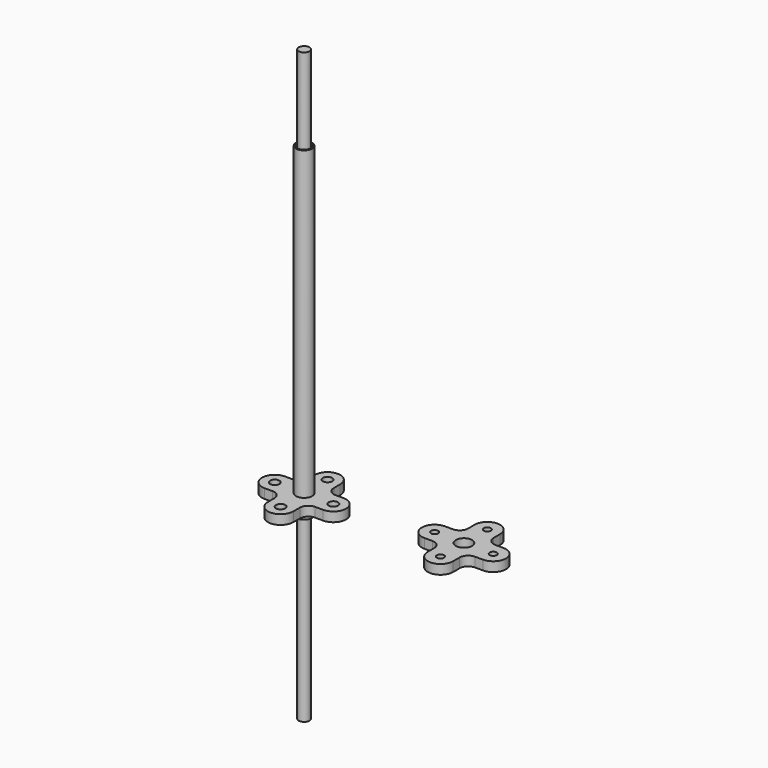
from build123d import *

# Parameters (mm, degrees)
F0_R          = 3.175
F1_DEPTH      = 235.8
F1_DEPTH_BACK = 111.4
F2_R          = 4.7625
F2_R_2        = 4.0259
F3_DEPTH      = 185.8
F3_DEPTH_BACK = 5.7
F4_R          = 2.75
F4_R_2        = 4.7625
F6_DEPTH      = 5.6
F5_R          = 2.1
F5_R_2        = 4.7625
F7_DEPTH      = 5.6


# Not quite as in the source:
# - ends of sketch curves that miss each other by under 0.0002 mm in the source are joined


with BuildPart() as f1:
    # F0 (on Top) → F1 (new body, two sides)
    with BuildSketch(Plane.XY) as f1_sk:
        Circle(F0_R)
    extrude(amount=F1_DEPTH)
    extrude(f1_sk.sketch, amount=-F1_DEPTH_BACK)


with BuildPart() as f3:
    # F2 (on Top) → F3 (new body, two sides)
    with BuildSketch(Plane.XY) as f3_sk:
        Circle(F2_R)
        Circle(F2_R_2, mode=Mode.SUBTRACT)
    extrude(amount=F3_DEPTH)
    extrude(f3_sk.sketch, amount=-F3_DEPTH_BACK)


with BuildPart() as f6:
    # F4 (on Top) → F6 (new body)
    with BuildSketch(Plane.XY):
        with BuildLine():
            ThreePointArc((7.5, 17.2625), (0, 24.7625), (-7.5, 17.2625))
            Line((-7.5, 17.2625), (-7.5, 12.5))
            ThreePointArc((-7.5, 12.5), (-8.9644660941, 8.9644660941), (-12.5, 7.5))
            Line((-12.5, 7.5), (-17.2627241709, 7.5))
            ThreePointArc((-17.2627241709, 7.5), (-22.5660250298, 5.3033008589), (-24.7627241709, 0))
            Line((-24.7627241709, 0), (-24.7626267772, -0.0382216857))
            ThreePointArc((-24.7626267772, -0.0382216857), (-22.5524943624, -5.3167970924), (-17.2627241709, -7.5))
            Line((-17.2627241709, -7.5), (-12.5, -7.5))
            ThreePointArc((-12.5, -7.5), (-8.9644660941, -8.9644660941), (-7.5, -12.5))
            Line((-7.5, -12.5), (-7.5, -17.2625))
            ThreePointArc((-7.5, -17.2625), (0, -24.7625), (7.5, -17.2625))
            Line((7.5, -17.2625), (7.5, -12.5))
            ThreePointArc((7.5, -12.5), (8.9644660941, -8.9644660941), (12.5, -7.5))
            Line((12.5, -7.5), (17.2625, -7.5))
            ThreePointArc((17.2625, -7.5), (24.7625, 0), (17.2625, 7.5))
            Line((17.2625, 7.5), (12.5, 7.5))
            ThreePointArc((12.5, 7.5), (8.9644660941, 8.9644660941), (7.5, 12.5))
            Line((7.5, 12.5), (7.5, 17.2625))
        make_face()
        with Locations((0, -17.2625)):
            Circle(F4_R, mode=Mode.SUBTRACT)
        with Locations((-17.2627241709, 0)):
            Circle(F4_R, mode=Mode.SUBTRACT)
        Circle(F4_R_2, mode=Mode.SUBTRACT)
        with Locations((17.2625, 0)):
            Circle(F4_R, mode=Mode.SUBTRACT)
        with Locations((0, 17.2625)):
            Circle(F4_R, mode=Mode.SUBTRACT)
    extrude(amount=F6_DEPTH)


with BuildPart() as f7:
    # F5 (on Top) → F7 (new body)
    with BuildSketch(Plane.XY):
        with BuildLine():
            ThreePointArc((95.9384369603, 24.4392953578), (88.4384369603, 31.9392953578), (80.9384369603, 24.4392953578))
            Line((80.9384369603, 24.4392953578), (80.9384369603, 19.6767953578))
            ThreePointArc((80.9384369603, 19.6767953578), (79.4739708663, 16.1412614519), (75.9384369603, 14.6767953578))
            Line((75.9384369603, 14.6767953578), (71.1757127894, 14.6767953578))
            ThreePointArc((71.1757127894, 14.6767953578), (65.8724119305, 12.4800962167), (63.6757127894, 7.1767953578))
            Line((63.6757127894, 7.1767953578), (63.6758101832, 7.1385736721))
            ThreePointArc((63.6758101832, 7.1385736721), (65.8859425979, 1.8599982654), (71.1757127894, -0.3232046422))
            Line((71.1757127894, -0.3232046422), (75.9384369603, -0.3232046422))
            ThreePointArc((75.9384369603, -0.3232046422), (79.4739708663, -1.7876707363), (80.9384369603, -5.3232046422))
            Line((80.9384369603, -5.3232046422), (80.9384369603, -10.0857046422))
            ThreePointArc((80.9384369603, -10.0857046422), (88.4384369603, -17.5857046422), (95.9384369603, -10.0857046422))
            Line((95.9384369603, -10.0857046422), (95.9384369603, -5.3232046422))
            ThreePointArc((95.9384369603, -5.3232046422), (97.4029030544, -1.7876707363), (100.9384369603, -0.3232046422))
            Line((100.9384369603, -0.3232046422), (105.7009369603, -0.3232046422))
            ThreePointArc((105.7009369603, -0.3232046422), (113.2009369603, 7.1767953578), (105.7009369603, 14.6767953578))
            Line((105.7009369603, 14.6767953578), (100.9384369603, 14.6767953578))
            ThreePointArc((100.9384369603, 14.6767953578), (97.4029030544, 16.1412614519), (95.9384369603, 19.6767953578))
            Line((95.9384369603, 19.6767953578), (95.9384369603, 24.4392953578))
        make_face()
        with Locations((71.1757127894, 7.1767953578)):
            Circle(F5_R, mode=Mode.SUBTRACT)
        with Locations((88.4384369603, -10.0857046422)):
            Circle(F5_R, mode=Mode.SUBTRACT)
        with Locations((88.4384369603, 7.1767953578)):
            Circle(F5_R_2, mode=Mode.SUBTRACT)
        with Locations((105.7009369603, 7.1767953578)):
            Circle(F5_R, mode=Mode.SUBTRACT)
        with Locations((88.4384369603, 24.4392953578)):
            Circle(F5_R, mode=Mode.SUBTRACT)
    extrude(amount=F7_DEPTH)


solid = Compound([f1.part, f3.part, f6.part, f7.part])
